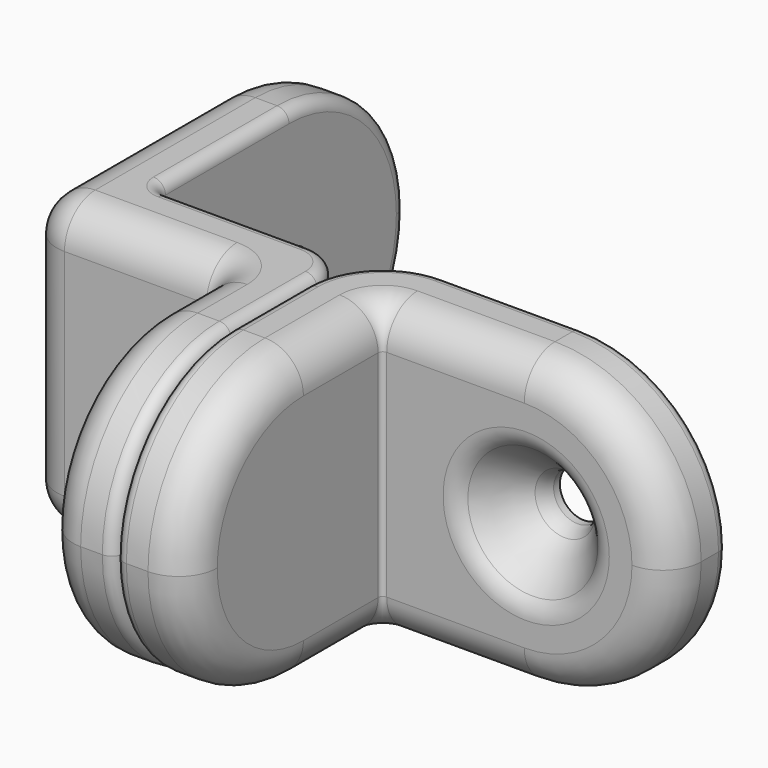
from build123d import *

# Parameters (mm, degrees)
F2_DEPTH     = 9.652
F3_DEPTH     = 9.652
F4_W         = 2.38125
F4_H         = 6.477
F10_R        = 9.65199
F10_2_R      = 9.65199
F11_R        = 9.65199
F11_2_R      = 9.65199
F12_T1_DEPTH = 44.704
F13_R        = 0.3175
F14_R        = 2.54
F15_R        = 2.54
F15_2_R      = 2.54
F16_R        = 0.79375
F17_R        = 0.79375
F17_2_R      = 0.79375
F18_R        = 1.5875
F18_2_R      = 1.5875
F19_R        = 2.54


# Not quite as in the source:
# - a fillet or chamfer that OpenCascade refuses, or shapes differently, is made with other operations: its cross-section is extruded or revolved along the edge and cut away or added
# - a fillet or chamfer is up to 0.001 mm smaller than in the source, because OpenCascade refuses the exact size


with BuildPart() as f2:
    # F0 (on Top) → F2 (new body, symmetric)
    with BuildSketch(Plane.XY):
        Polygon((0, -1.5875), (0, 19.05), (-4.7625, 19.05), (-4.7625, -6.35), (7.9375, -6.35), (7.9375, -20.8915), (12.7, -20.8915), (12.7, -1.5875), align=None)
    extrude(amount=F2_DEPTH, both=True)


with BuildPart() as f3:
    # F1 (on Top) → F3 (new body, symmetric)
    with BuildSketch(Plane.XY):
        Polygon((36.5125, 0), (12.7, 0), (12.7, -20.8915), (17.4625, -20.8915), (17.4625, -4.7625), (36.5125, -4.7625), align=None)
    extrude(amount=F3_DEPTH, both=True)


with BuildPart() as f5_tool:
    # F4 (on Top) → F5 (revolve)
    with BuildSketch(Plane.XY):
        with Locations((12.7, -8.001)):
            Rectangle(F4_W, F4_H)
    revolve(axis=Axis((19.7726818566, -11.2395, 0), (1, 0, 0)))


with BuildPart() as f2_1:
    add(f2.part)

    # F5: cut by f5_tool
    add(f5_tool.part, mode=Mode.SUBTRACT)

    # F6 (on Top) → F7 (revolve, cut)
    with BuildSketch(Plane.XY):
        Polygon((-1.1100803071, 11.1125), (-4.7625, 14.2875), (-4.7625, 9.525), (0, 9.525), (0, 11.1125), align=None)
    revolve(axis=Axis((4.3882697649, 9.525, 0), (1, 0, 0)), mode=Mode.SUBTRACT)

    # F10 (radius 9.652 in the source; OpenCascade refuses exactly that, so slightly less here)
    f10_edges = [f2_1.edges().sort_by_distance(p)[0] for p in [
        (10.31875, -20.8915, 9.652),
        (10.31875, -20.8915, -9.652),
    ]]
    fillet(f10_edges, radius=F10_R)

    # F11 (radius 9.652 in the source; OpenCascade refuses exactly that, so slightly less here)
    f11_edges = [f2_1.edges().sort_by_distance(p)[0] for p in [
        (-2.38125, 19.05, 9.652),
        (-2.38125, 19.05, -9.652),
    ]]
    fillet(f11_edges, radius=F11_R)

    # F14
    f14_edges = [f2_1.edges().sort_by_distance(p)[0] for p in [
        (12.7, -1.5875, 0),
    ]]
    fillet(f14_edges, radius=F14_R)

    # F15
    f15_edges = [f2_1.edges().sort_by_distance(p)[0] for p in [
        (-4.7625, 1.524005, 9.652),
    ]]
    fillet(f15_edges, radius=F15_R)

    # F16
    f16_edges = [f2_1.edges().sort_by_distance(p)[0] for p in [
        (0, -1.5875, 0),
        (7.9375, -6.35, 0),
    ]]
    fillet(f16_edges, radius=F16_R)

    # F17
    f17_edges = [f2_1.edges().sort_by_distance(p)[0] for p in [
        (0, 4.30213, 9.652),
        (0, 4.30213, -9.652),
        (0.232484, -1.355016, -9.652),
        (5.476875, -1.5875, -9.652),
        (11.956051, -2.331449, -9.652),
        (12.7, -7.683505, -9.652),
        (0, 16.222998, -6.824998),
        (0, 19.05, 0),
        (0, 16.222998, 6.824998),
        (0.232484, -1.355016, 9.652),
        (5.476875, -1.5875, 9.652),
        (11.956051, -2.331449, 9.652),
        (12.7, -18.064498, -6.824998),
        (12.7, -7.683505, 9.652),
        (12.7, -20.8915, 0),
        (12.7, -18.064498, 6.824998),
    ]]
    fillet(f17_edges, radius=F17_R)

    # F18
    f18_edges = [f2_1.edges().sort_by_distance(p)[0] for p in [
        (-4.7625, 4.7625, 0),
        (-1.11008, 7.9375, 0),
    ]]
    fillet(f18_edges, radius=F18_R)

    # F19
    f19_edges = [f2_1.edges().sort_by_distance(p)[0] for p in [
        (2.460625, -6.35, 9.652),
        (-4.7625, -6.35, 0),
        (2.460625, -6.35, -9.652),
        (-4.018551, -6.35, -8.908051),
        (-4.018551, -6.35, 8.908051),
        (7.705016, -6.582484, -9.652),
        (7.9375, -9.19163, -9.652),
        (7.705016, -6.582484, 9.652),
        (7.9375, -9.19163, 9.652),
        (7.9375, -18.064498, -6.824998),
        (7.9375, -20.8915, 0),
        (7.9375, -18.064498, 6.824998),
    ]]
    fillet(f19_edges, radius=F19_R)


with BuildPart() as f3_1:
    add(f3.part)

    # F5: cut by f5_tool
    add(f5_tool.part, mode=Mode.SUBTRACT)

    # F8 (on Top) → F9 (revolve, cut)
    with BuildSketch(Plane.XY):
        Polygon((28.575, -1.1100803071), (28.575, 0), (26.9875, 0), (26.9875, -4.7625), (31.75, -4.7625), align=None)
    revolve(axis=Axis((26.9875, 5.8666377451, 0), (0, 1, 0)), mode=Mode.SUBTRACT)

    # F10#2 (radius 9.652 in the source; OpenCascade refuses exactly that, so slightly less here)
    f10_2_edges = [f3_1.edges().sort_by_distance(p)[0] for p in [
        (15.08125, -20.8915, 9.652),
        (15.08125, -20.8915, -9.652),
    ]]
    fillet(f10_2_edges, radius=F10_2_R)

    # F11#2 (radius 9.652 in the source; OpenCascade refuses exactly that, so slightly less here)
    f11_2_edges = [f3_1.edges().sort_by_distance(p)[0] for p in [
        (36.5125, -2.38125, 9.652),
        (36.5125, -2.38125, -9.652),
    ]]
    fillet(f11_2_edges, radius=F11_2_R)

    # F12: fillet of radius 5.08 on 1 edges, made by hand

    # F12_s2 → F12_t1 (cut)
    with BuildSketch(Plane.XY.offset(-22.352)):
        with BuildLine():
            ThreePointArc((17.78, 0), (14.1878975516, -1.4878975516), (12.7, -5.08))
            Line((12.7, -5.08), (12.7, 0))
            Line((12.7, 0), (17.78, 0))
        make_face()
    extrude(amount=F12_T1_DEPTH, mode=Mode.SUBTRACT)

    # F13
    f13_edges = [f3_1.edges().sort_by_distance(p)[0] for p in [
        (17.4625, -4.7625, 0),
    ]]
    fillet(f13_edges, radius=F13_R)

    # F15#2
    f15_2_edges = [f3_1.edges().sort_by_distance(p)[0] for p in [
        (22.320255, -4.7625, 9.652),
    ]]
    fillet(f15_2_edges, radius=F15_2_R)

    # F17#2
    f17_2_edges = [f3_1.edges().sort_by_distance(p)[0] for p in [
        (22.320255, 0, 9.652),
        (12.7, -18.064498, -6.824998),
        (12.7, -20.8915, 0),
        (12.7, -18.064498, 6.824998),
        (22.320255, 0, -9.652),
        (14.187898, -1.487898, -9.652),
        (12.7, -8.159755, -9.652),
        (33.685498, 0, -6.824998),
        (36.5125, 0, 0),
        (33.685498, 0, 6.824998),
        (14.187898, -1.487898, 9.652),
        (12.7, -8.159755, 9.652),
    ]]
    fillet(f17_2_edges, radius=F17_2_R)

    # F18#2
    f18_2_edges = [f3_1.edges().sort_by_distance(p)[0] for p in [
        (22.225, -4.7625, 0),
        (25.4, -1.11008, 0),
    ]]
    fillet(f18_2_edges, radius=F18_2_R)


solid = Compound([f2_1.part, f3_1.part])
